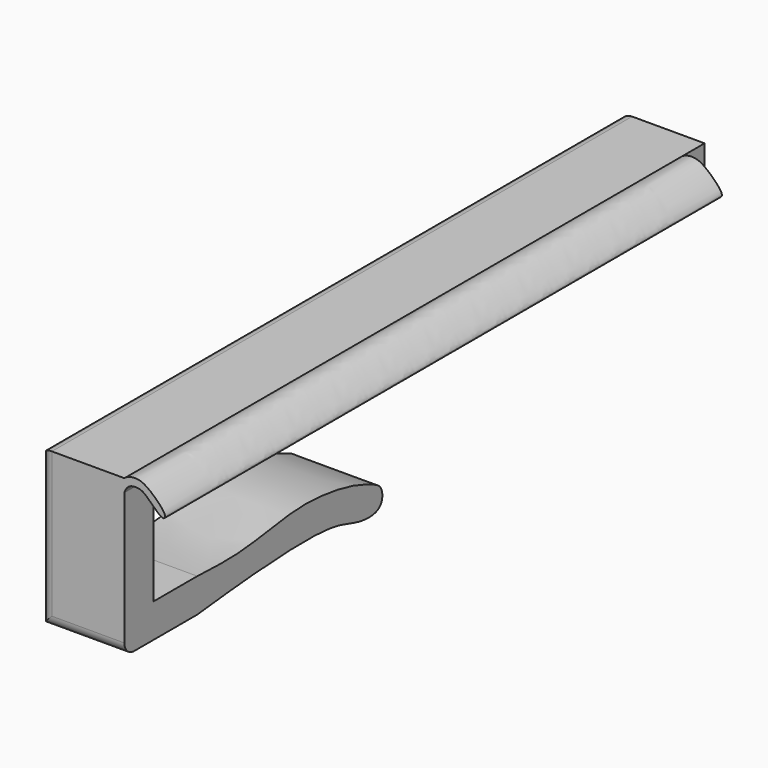
from build123d import *

# Parameters (mm, degrees)
F0_W     = 144.78
F0_H     = 6.35
F0_W_2   = 11.5199978839
F0_H_2   = 7.112
F1_DEPTH = 17.78
F3_DEPTH = 146.25322
F4_R     = 2.54


with BuildPart() as f1:
    # F0 (on Right) → F1 (new body)
    with BuildSketch(Plane.YZ):
        Polygon((7.62, 0), (0, 0), (0, -33.02), (7.62, -33.02), (7.62, -25.908), (7.62, -6.35), align=None)
        with Locations((80.01, -3.175)):
            Rectangle(F0_W, F0_H)
        with Locations((13.379998942, -29.464)):
            Rectangle(F0_W_2, F0_H_2)
        with BuildLine():
            Line((19.1399978839, -25.908), (19.1399978839, -33.02))
            add(Edge.make_bspline(
                [(19.1399978839, -25.908), (22.6205993471, -26.0265720278), (31.7393433845, -26.5846352029), (46.426421665, -23.0401959905), (60.2469922652, -25.5316489193), (64.2200697328, -27.3919290244), (68.0270994306, -28.6765434409), (67.8018861653, -33.848544154), (56.094779184, -32.877209402), (55.5899702013, -28.9649087936), (19.1399978839, -33.02)],
                knots=[0, 0, 0, 0, 0.1350742157, 0.2893317868, 0.4314811015, 0.5125951644, 0.5842753079, 0.6555688227, 0.7486551591, 1, 1, 1, 1], degree=3))
        make_face()
    extrude(amount=F1_DEPTH)

    # F2 (on face) → F3 (join)
    with BuildSketch(Plane.XZ):
        with BuildLine():
            add(Edge.make_bspline(
                [(17.78, 0), (18.1444263839, 0.3479734295), (19.125747791, 0.7060246273), (20.0914297681, 0.7764735174), (20.8218672984, 0.6663874974), (22.4488839757, 0.3146673841), (26.9319247263, -3.8838589536), (25.8581610742, -5.1602741578), (23.8281447001, -3.1722776308), (22.5226644895, -1.9010419247), (21.317845023, -0.9044466981), (19.4197732241, -0.7966284026), (18.2752425961, -1.4649505679), (17.8322992215, -2.4109045487), (17.78, -2.6894505136)],
                knots=[0, 0, 0, 0, 0.0749092424, 0.1341411687, 0.1825874628, 0.2630487514, 0.4085586112, 0.4592612339, 0.5549422291, 0.6412908922, 0.7151009854, 0.7958994616, 0.86540537, 0.9322690578, 0.9322690578, 0.9322690578, 0.9322690578], degree=3))
            Line((17.78, 0), (17.78, -2.6894505136))
        make_face()
    extrude(amount=-F3_DEPTH)

    # F4
    f4_edges = [f1.edges().sort_by_distance(p)[0] for p in [
        (0, 76.2, 0),
        (8.89, 0, -33.02),
        (0, 0, -16.51),
    ]]
    fillet(f4_edges, radius=F4_R)


solid = f1.part
